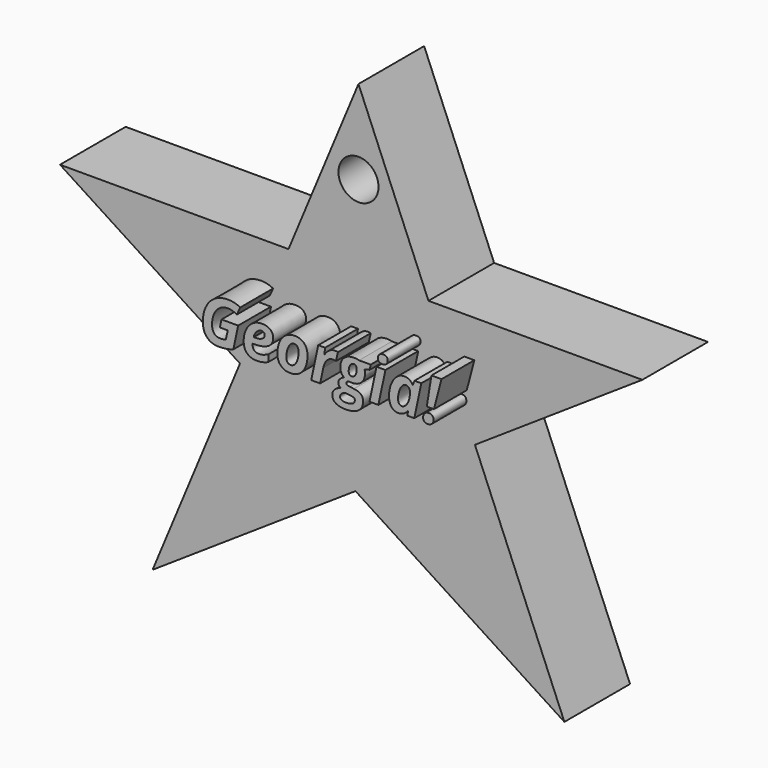
from build123d import *

# Parameters (mm, degrees)
F1_DEPTH     = 10
F2_TEXT_SIZE = 7.3780886139
F3_DEPTH     = 5
F4_R         = 2.4409406921
F5_DEPTH     = 10.001


# Not quite as in the source:
# - Text() gives the source's letters only with a copy of the font that has no kerning and outlines rounded to 1/6400 em; it was checked with that copy


with BuildPart() as f1:
    # F0 (on Front) → F1 (new body)
    with BuildSketch(Plane.XZ):
        Polygon((-14.4392097673, 13.5637482204), (-25.0910539436, -12.025889669), (-0.3689855723, 4.4554876532), (25.0910539436, -12.025889669), (14.1903142421, 14.1616865919), (34.5929945678, 27.7634721618), (8.5284873325, 27.7634721618), (0, 48.2520278494), (-8.5284873325, 27.7634721618), (-36.3746054322, 27.7634721618), align=None)
    extrude(amount=F1_DEPTH)

    # F2 (on face) → F3 (join)
    with BuildSketch(Plane.XZ.offset(10)):
        with Locations((-15.4069075997, 17.9398040474)):
            Text('Georgia!', F2_TEXT_SIZE, font='Open Sans', font_style=FontStyle.BOLDITALIC, text_align=(TextAlign.LEFT, TextAlign.BOTTOM))
    extrude(amount=F3_DEPTH)

    # F4 (on face) → F5 (cut, through all)
    with BuildSketch(Plane.XZ.offset(10)):
        with Locations((0, 38.0077500056)):
            Circle(F4_R)
    extrude(amount=-F5_DEPTH, mode=Mode.SUBTRACT)


solid = f1.part
